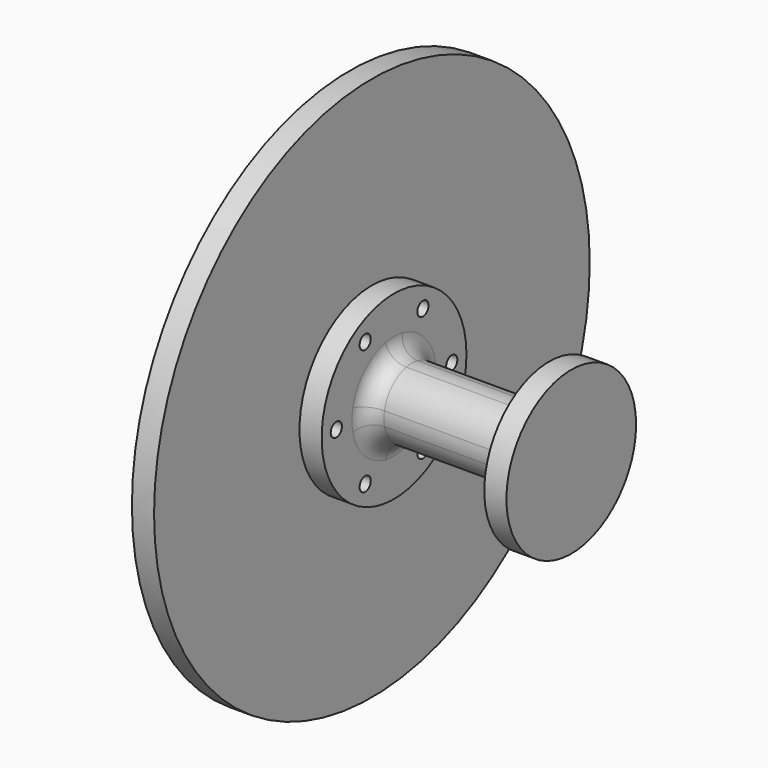
from build123d import *

# Parameters (mm, degrees)
F0_W       = 6
F0_H       = 4
F0_W_2     = 4
F0_H_2     = 6
F1_DEPTH   = 50.8
F0_R       = 25.9436510784
F2_DEPTH   = 6.35
F3_R       = 78.0540986602
F3_R_2     = 25.9436510784
F4_DEPTH   = 6.35
F5_R       = 23.2299386705
F5_W       = 4
F5_H       = 6
F5_W_2     = 6
F5_H_2     = 4
F6_DEPTH   = 6.35
F7_R       = 5.08
F8_D       = 4
F8_DEPTH   = 57.151
F8_2_D     = 4
F8_2_DEPTH = 57.151


with BuildPart() as f1:
    # F0 (on Right) → F1 (new body)
    with BuildSketch(Plane.YZ):
        with BuildLine():
            ThreePointArc((2, -9.7979589711), (7.0710678119, -7.0710678119), (9.7979589711, -2))
            Line((9.7979589711, -2), (8, -2))
            Line((8, -2), (2, -2))
            Line((2, -2), (2, -8))
            Line((2, -8), (2, -9.7979589711))
        make_face()
        with BuildLine():
            ThreePointArc((-9.7979589711, -2), (-7.0710678119, -7.0710678119), (-2, -9.7979589711))
            Line((-2, -9.7979589711), (-2, -8))
            Line((-2, -8), (-2, -2))
            Line((-2, -2), (-8, -2))
            Line((-8, -2), (-9.7979589711, -2))
        make_face()
        with BuildLine():
            Line((-2, 8), (-2, 9.7979589711))
            ThreePointArc((-2, 9.7979589711), (-7.0710678119, 7.0710678119), (-9.7979589711, 2))
            Line((-9.7979589711, 2), (-8, 2))
            Line((-8, 2), (-2, 2))
            Line((-2, 2), (-2, 8))
        make_face()
        with BuildLine():
            Line((8, 2), (9.7979589711, 2))
            ThreePointArc((9.7979589711, 2), (7.0710678119, 7.0710678119), (2, 9.7979589711))
            Line((2, 9.7979589711), (2, 8))
            Line((2, 8), (2, 2))
            Line((2, 2), (8, 2))
        make_face()
        with Locations((5, 0)):
            Rectangle(F0_W, F0_H)
        Rectangle(F0_W_2, F0_H)
        with Locations((0, 5)):
            Rectangle(F0_W_2, F0_H_2)
        with Locations((-5, 0)):
            Rectangle(F0_W, F0_H)
        with Locations((0, -5)):
            Rectangle(F0_W_2, F0_H_2)
        with BuildLine():
            Line((-8, 2), (-9.7979589711, 2))
            ThreePointArc((-9.7979589711, 2), (-10, 0), (-9.7979589711, -2))
            Line((-9.7979589711, -2), (-8, -2))
            Line((-8, -2), (-8, 2))
        make_face()
        with BuildLine():
            ThreePointArc((-2, -9.7979589711), (0, -10), (2, -9.7979589711))
            Line((2, -9.7979589711), (2, -8))
            Line((2, -8), (-2, -8))
            Line((-2, -8), (-2, -9.7979589711))
        make_face()
        with BuildLine():
            ThreePointArc((9.7979589711, -2), (9.9493615301, -1.0050896201), (10, 0))
            ThreePointArc((10, 0), (9.9493615301, 1.0050896201), (9.7979589711, 2))
            Line((9.7979589711, 2), (8, 2))
            Line((8, 2), (8, -2))
            Line((8, -2), (9.7979589711, -2))
        make_face()
        with BuildLine():
            Line((2, 8), (2, 9.7979589711))
            ThreePointArc((2, 9.7979589711), (0, 10), (-2, 9.7979589711))
            Line((-2, 9.7979589711), (-2, 8))
            Line((-2, 8), (2, 8))
        make_face()
    extrude(amount=F1_DEPTH)

    # F0 (on Right) → F2 (join)
    with BuildSketch(Plane.YZ):
        Circle(F0_R)
        Polygon((10.3425991178, 17.9139071543), (20.6851982355, 0), (10.3425991178, -17.9139071543), (-10.3425991178, -17.9139071543), (-20.6851982355, 0), (-10.3425991178, 17.9139071543), align=None, mode=Mode.SUBTRACT)
        Polygon((10.3425991178, -17.9139071543), (20.6851982355, 0), (10.3425991178, 17.9139071543), (-10.3425991178, 17.9139071543), (-20.6851982355, 0), (-10.3425991178, -17.9139071543), align=None)
        with BuildLine():
            ThreePointArc((2, 9.7979589711), (7.0710678119, 7.0710678119), (9.7979589711, 2))
            Line((9.7979589711, 2), (12.5, 2))
            Line((12.5, 2), (12.5, -2))
            Line((12.5, -2), (9.7979589711, -2))
            ThreePointArc((9.7979589711, -2), (7.0710678119, -7.0710678119), (2, -9.7979589711))
            Line((2, -9.7979589711), (2, -12.5))
            Line((2, -12.5), (-2, -12.5))
            Line((-2, -12.5), (-2, -9.7979589711))
            ThreePointArc((-2, -9.7979589711), (-7.0710678119, -7.0710678119), (-9.7979589711, -2))
            Line((-9.7979589711, -2), (-12.5, -2))
            Line((-12.5, -2), (-12.5, 2))
            Line((-12.5, 2), (-9.7979589711, 2))
            ThreePointArc((-9.7979589711, 2), (-7.0710678119, 7.0710678119), (-2, 9.7979589711))
            Line((-2, 9.7979589711), (-2, 12.5))
            Line((-2, 12.5), (2, 12.5))
            Line((2, 12.5), (2, 9.7979589711))
        make_face(mode=Mode.SUBTRACT)
        with BuildLine():
            ThreePointArc((-2, 9.7979589711), (0, 10), (2, 9.7979589711))
            Line((2, 9.7979589711), (2, 12.5))
            Line((2, 12.5), (-2, 12.5))
            Line((-2, 12.5), (-2, 9.7979589711))
        make_face()
        with BuildLine():
            ThreePointArc((9.7979589711, 2), (9.9493615301, 1.0050896201), (10, 0))
            ThreePointArc((10, 0), (9.9493615301, -1.0050896201), (9.7979589711, -2))
            Line((9.7979589711, -2), (12.5, -2))
            Line((12.5, -2), (12.5, 2))
            Line((12.5, 2), (9.7979589711, 2))
        make_face()
        with BuildLine():
            ThreePointArc((-9.7979589711, -2), (-10, 0), (-9.7979589711, 2))
            Line((-9.7979589711, 2), (-12.5, 2))
            Line((-12.5, 2), (-12.5, -2))
            Line((-12.5, -2), (-9.7979589711, -2))
        make_face()
        with BuildLine():
            Line((2, -12.5), (2, -9.7979589711))
            ThreePointArc((2, -9.7979589711), (0, -10), (-2, -9.7979589711))
            Line((-2, -9.7979589711), (-2, -12.5))
            Line((-2, -12.5), (2, -12.5))
        make_face()
    extrude(amount=F2_DEPTH)

    # F5 (on face) → F6 (join)
    with BuildSketch(Plane.YZ.offset(50.8)):
        Circle(F5_R)
        Polygon((10.3425991178, 17.9139071543), (20.6851982355, 0), (10.3425991178, -17.9139071543), (-10.3425991178, -17.9139071543), (-20.6851982355, 0), (-10.3425991178, 17.9139071543), align=None, mode=Mode.SUBTRACT)
        Polygon((10.3425991178, -17.9139071543), (20.6851982355, 0), (10.3425991178, 17.9139071543), (-10.3425991178, 17.9139071543), (-20.6851982355, 0), (-10.3425991178, -17.9139071543), align=None)
        with BuildLine():
            ThreePointArc((2, 9.7979589711), (7.0710678119, 7.0710678119), (9.7979589711, 2))
            Line((9.7979589711, 2), (12.5, 2))
            Line((12.5, 2), (12.5, -2))
            Line((12.5, -2), (9.7979589711, -2))
            ThreePointArc((9.7979589711, -2), (7.0710678119, -7.0710678119), (2, -9.7979589711))
            Line((2, -9.7979589711), (2, -12.5))
            Line((2, -12.5), (-2, -12.5))
            Line((-2, -12.5), (-2, -9.7979589711))
            ThreePointArc((-2, -9.7979589711), (-7.0710678119, -7.0710678119), (-9.7979589711, -2))
            Line((-9.7979589711, -2), (-12.5, -2))
            Line((-12.5, -2), (-12.5, 2))
            Line((-12.5, 2), (-9.7979589711, 2))
            ThreePointArc((-9.7979589711, 2), (-7.0710678119, 7.0710678119), (-2, 9.7979589711))
            Line((-2, 9.7979589711), (-2, 12.5))
            Line((-2, 12.5), (2, 12.5))
            Line((2, 12.5), (2, 9.7979589711))
        make_face(mode=Mode.SUBTRACT)
        with BuildLine():
            Line((8, 2), (9.7979589711, 2))
            ThreePointArc((9.7979589711, 2), (7.0710678119, 7.0710678119), (2, 9.7979589711))
            Line((2, 9.7979589711), (2, 8))
            Line((2, 8), (2, 2))
            Line((2, 2), (8, 2))
        make_face()
        with BuildLine():
            ThreePointArc((2, -9.7979589711), (7.0710678119, -7.0710678119), (9.7979589711, -2))
            Line((9.7979589711, -2), (8, -2))
            Line((8, -2), (2, -2))
            Line((2, -2), (2, -8))
            Line((2, -8), (2, -9.7979589711))
        make_face()
        with BuildLine():
            ThreePointArc((-9.7979589711, -2), (-7.0710678119, -7.0710678119), (-2, -9.7979589711))
            Line((-2, -9.7979589711), (-2, -8))
            Line((-2, -8), (-2, -2))
            Line((-2, -2), (-8, -2))
            Line((-8, -2), (-9.7979589711, -2))
        make_face()
        with BuildLine():
            Line((-2, 8), (-2, 9.7979589711))
            ThreePointArc((-2, 9.7979589711), (-7.0710678119, 7.0710678119), (-9.7979589711, 2))
            Line((-9.7979589711, 2), (-8, 2))
            Line((-8, 2), (-2, 2))
            Line((-2, 2), (-2, 8))
        make_face()
        with Locations((0, 5)):
            Rectangle(F5_W, F5_H)
        with Locations((5, 0)):
            Rectangle(F5_W_2, F5_H_2)
        with Locations((0, -5)):
            Rectangle(F5_W, F5_H)
        with Locations((-5, 0)):
            Rectangle(F5_W_2, F5_H_2)
        Rectangle(F5_W, F5_H_2)
        with BuildLine():
            ThreePointArc((-2, 9.7979589711), (0, 10), (2, 9.7979589711))
            Line((2, 9.7979589711), (2, 12.5))
            Line((2, 12.5), (-2, 12.5))
            Line((-2, 12.5), (-2, 9.7979589711))
        make_face()
        with BuildLine():
            ThreePointArc((9.7979589711, 2), (9.9493615301, 1.0050896201), (10, 0))
            ThreePointArc((10, 0), (9.9493615301, -1.0050896201), (9.7979589711, -2))
            Line((9.7979589711, -2), (12.5, -2))
            Line((12.5, -2), (12.5, 2))
            Line((12.5, 2), (9.7979589711, 2))
        make_face()
        with BuildLine():
            Line((2, -12.5), (2, -9.7979589711))
            ThreePointArc((2, -9.7979589711), (0, -10), (-2, -9.7979589711))
            Line((-2, -9.7979589711), (-2, -12.5))
            Line((-2, -12.5), (2, -12.5))
        make_face()
        with BuildLine():
            ThreePointArc((-9.7979589711, -2), (-10, 0), (-9.7979589711, 2))
            Line((-9.7979589711, 2), (-12.5, 2))
            Line((-12.5, 2), (-12.5, -2))
            Line((-12.5, -2), (-9.7979589711, -2))
        make_face()
        with BuildLine():
            Line((2, 8), (2, 9.7979589711))
            ThreePointArc((2, 9.7979589711), (0, 10), (-2, 9.7979589711))
            Line((-2, 9.7979589711), (-2, 8))
            Line((-2, 8), (2, 8))
        make_face()
        with BuildLine():
            ThreePointArc((9.7979589711, -2), (9.9493615301, -1.0050896201), (10, 0))
            ThreePointArc((10, 0), (9.9493615301, 1.0050896201), (9.7979589711, 2))
            Line((9.7979589711, 2), (8, 2))
            Line((8, 2), (8, -2))
            Line((8, -2), (9.7979589711, -2))
        make_face()
        with BuildLine():
            ThreePointArc((-2, -9.7979589711), (0, -10), (2, -9.7979589711))
            Line((2, -9.7979589711), (2, -8))
            Line((2, -8), (-2, -8))
            Line((-2, -8), (-2, -9.7979589711))
        make_face()
        with BuildLine():
            Line((-8, 2), (-9.7979589711, 2))
            ThreePointArc((-9.7979589711, 2), (-10, 0), (-9.7979589711, -2))
            Line((-9.7979589711, -2), (-8, -2))
            Line((-8, -2), (-8, 2))
        make_face()
    extrude(amount=F6_DEPTH)

    # F7
    f7_edges = [f1.edges().sort_by_distance(p)[0] for p in [
        (6.35, -2, -9.797959),
    ]]
    fillet(f7_edges, radius=F7_R)

    # F8 (through all, one way)
    with BuildSketch(Plane.YZ.offset(50.8)):
        with Locations((10.3425991178, 17.9139071543), (20.6851982355, 0), (-10.3425991178, 17.9139071543), (10.3425991178, -17.9139071543), (-10.3425991178, -17.9139071543), (-20.6851982355, 0)):
            Circle(F8_D / 2)
    extrude(amount=-F8_DEPTH, mode=Mode.SUBTRACT)


with BuildPart() as f4:
    # F3 (on face) → F4 (new body)
    with BuildSketch(Plane(origin=(0, 0, 0), x_dir=(0, -1, 0), z_dir=(-1, 0, 0))):
        Circle(F3_R)
        Circle(F3_R_2, mode=Mode.SUBTRACT)
        Circle(F3_R_2)
    extrude(amount=F4_DEPTH)

    # F8#2 (through all, one way)
    with BuildSketch(Plane.YZ.offset(50.8)):
        with Locations((10.3425991178, 17.9139071543), (20.6851982355, 0), (-10.3425991178, 17.9139071543), (10.3425991178, -17.9139071543), (-10.3425991178, -17.9139071543), (-20.6851982355, 0)):
            Circle(F8_2_D / 2)
    extrude(amount=-F8_2_DEPTH, mode=Mode.SUBTRACT)


solid = Compound([f1.part, f4.part])
